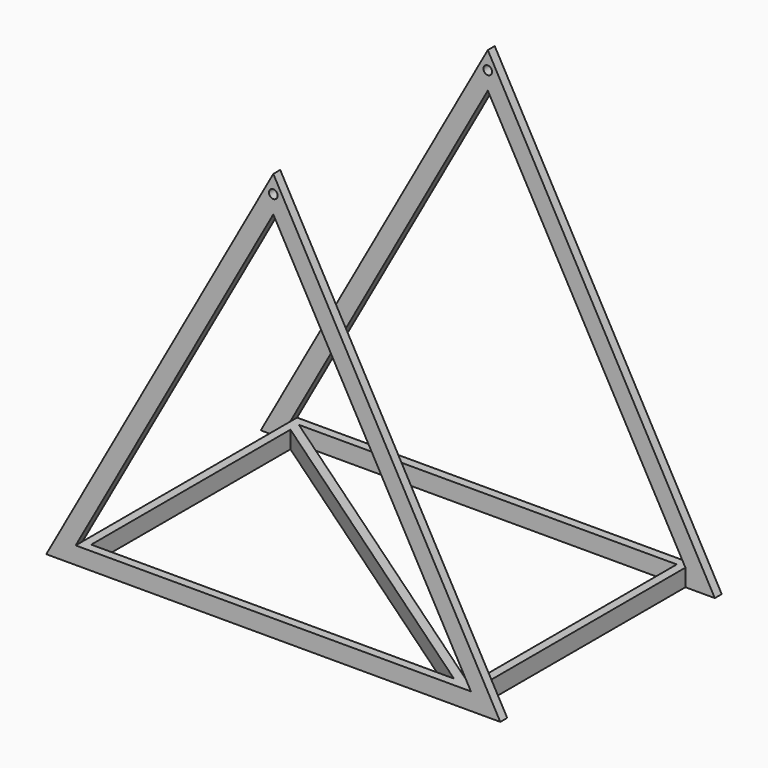
from build123d import *

# Parameters (mm, degrees)
F1_DEPTH = 19.05
F2_DEPTH = 19.05
F3_R     = 9.525
F4_DEPTH = 25
F5_W     = 19.05
F5_H     = 38.1
F6_DEPTH = 285.75
F9_DEPTH = 38.1


# Not quite as in the source:
# - a feature names something its author has since deleted; it is built from what else it names


with BuildPart() as f1:
    # F0 (on Front) → F1 (new body)
    with BuildSketch(Plane.XZ):
        Polygon((435.2484990698, 38.1), (-435.2484990698, 38.1), (-456.4151657365, 0), (456.4151657365, 0), align=None)
    extrude(amount=F1_DEPTH)

    # F0 (on Front) → F2 (join)
    with BuildSketch(Plane.XZ):
        Polygon((500, 0), (478.8333333333, 38.1), (435.2484990698, 38.1), (456.4151657365, 0), align=None)
        Polygon((478.8333333333, 38.1), (21.7924171318, 860.7736491628), (0, 821.5472983257), (435.2484990698, 38.1), align=None)
        Polygon((21.7924171318, 860.7736491628), (0, 900), (-21.7924171318, 860.7736491628), (0, 821.5472983257), align=None)
        Polygon((0, 821.5472983257), (-21.7924171318, 860.7736491628), (-478.8333333333, 38.1), (-435.2484990698, 38.1), align=None)
        Polygon((-435.2484990698, 38.1), (-478.8333333333, 38.1), (-500, 0), (-456.4151657365, 0), align=None)
    extrude(amount=F2_DEPTH)

    # F3 (on face) → F4 (cut)
    with BuildSketch(Plane.XZ.offset(19.05)):
        with Locations((0, 860.7736491628)):
            Circle(F3_R)
    extrude(amount=-F4_DEPTH, mode=Mode.SUBTRACT)

    # F5 (on face) → F6 (join)
    with BuildSketch(Plane.XZ.offset(19.05)):
        with Locations((-425.7234990698, 19.05)):
            Rectangle(F5_W, F5_H)
        with Locations((425.7234990698, 19.05)):
            Rectangle(F5_W, F5_H)
    extrude(amount=F6_DEPTH)

    # F7: F1 across face


with BuildPart() as f1_1:
    add(f1.part)
    add(f1.part.mirror(Plane(origin=(425.7234990698, -304.8, 19.05), x_dir=(1, 0, 0), z_dir=(0, -1, 0))))

    # F8 (on Top) → F9 (join, through all)
    with BuildSketch(Plane.XY):
        Polygon((416.1984990698, -590.55), (-416.1984990698, -19.05), (-416.1984990698, -42.1577389905), (382.5417841626, -590.55), align=None)
    extrude(amount=F9_DEPTH)


solid = f1_1.part
